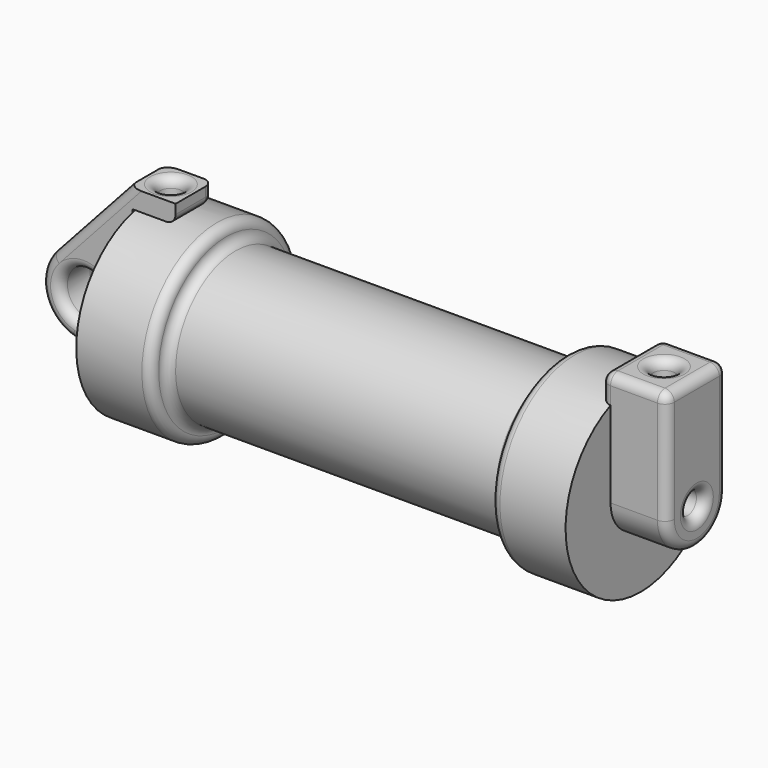
from build123d import *

# Parameters (mm, degrees)
F0_W            = 5.842
F0_H            = 12.7
F0_R            = 3.175
F2_DEPTH        = 3.175
F3_R            = 1.524
F4_DEPTH        = 7.62
F4_DEPTH_BACK   = 1.27
F5_DEPTH        = 56.134
F6_R            = 1.524
F7_DEPTH        = 10.414
F8_R            = 1.524
F9_DEPTH        = 17.78
F10_F1_R        = 1.27
F10_F2_R        = 1.2699
F10_2_T1_DEPTH  = 18.5821257943
F10_2_T3_DEPTH  = 4.572
F10_2_T5_DEPTH  = 4.445
F10_2_T7_DEPTH  = 8.255
F10_2_T9_DEPTH  = 17.7294216388
F10_2_S13_W     = 1.27
F10_2_S13_H     = 1.27
F10_2_T14_DEPTH = 1.27
F10_2_T20_ANGLE = 116.8111069241
F10_2_T26_ANGLE = 116.8111069241


# Not quite as in the source:
# - a fillet or chamfer that OpenCascade refuses, or shapes differently, is made with other operations: its cross-section is extruded or revolved along the edge and cut away or added
# - a fillet or chamfer is up to 0.001 mm smaller than in the source, because OpenCascade refuses the exact size


with BuildPart() as f1:
    # F0 (on Front) → F1 (revolve)
    with BuildSketch(Plane.XZ):
        with Locations((2.921, 6.35)):
            Rectangle(F0_W, F0_H)
        Polygon((5.842, 12.7), (5.842, 0), (66.294, 0), (66.294, 12.7), (56.134, 12.7), (56.134, 10.16), (10.16, 10.16), (10.16, 12.7), align=None)
    revolve(axis=Axis((33.147, 0, 0), (-1, 0, 0)))

    # F3 (on face) → F4 (join, two sides)
    with BuildSketch(Plane.YZ.offset(66.294)) as f4_sk:
        with BuildLine():
            ThreePointArc((-5.08, 0), (0, 5.08), (5.08, 0))
            Line((5.08, 0), (5.08, 11.6397422652))
            ThreePointArc((5.08, 11.6397422652), (0, 12.7), (-5.08, 11.6397422652))
            Line((-5.08, 11.6397422652), (-5.08, 0))
        make_face()
        with BuildLine():
            ThreePointArc((-5.08, 0), (0, -5.08), (5.08, 0))
            ThreePointArc((5.08, 0), (0, 5.08), (-5.08, 0))
        make_face()
        Circle(F3_R, mode=Mode.SUBTRACT)
        with BuildLine():
            ThreePointArc((-5.08, 11.6397422652), (0, 12.7), (5.08, 11.6397422652))
            Line((5.08, 11.6397422652), (5.08, 15.24))
            Line((5.08, 15.24), (-5.08, 15.24))
            Line((-5.08, 15.24), (-5.08, 11.6397422652))
        make_face()
    extrude(amount=F4_DEPTH)
    extrude(f4_sk.sketch, amount=-F4_DEPTH_BACK)

    # F3 (on face) → F5 (cut, through all)
    with BuildSketch(Plane.YZ.offset(66.294)):
        Circle(F3_R)
    extrude(amount=-F5_DEPTH, mode=Mode.SUBTRACT)

    # F6 (on face) → F7 (cut)
    with BuildSketch(Plane.XY.offset(15.24)):
        with Locations((69.469, 0)):
            Circle(F6_R)
    extrude(amount=-F7_DEPTH, mode=Mode.SUBTRACT)


with BuildPart() as f2:
    # F0 (on Front) → F2 (new body, symmetric)
    with BuildSketch(Plane.XZ):
        with BuildLine():
            Line((-0.9398, 0), (0, 0))
            Line((0, 0), (0, 12.7))
            Line((0, 12.7), (5.842, 12.7))
            Line((5.842, 12.7), (5.842, 15.24))
            Line((5.842, 15.24), (-0.508, 15.24))
            Line((-0.508, 15.24), (-10.8806298187, 3.8475430269))
            ThreePointArc((-10.8806298187, 3.8475430269), (-4.5919612295, 5.3297205562), (-0.9398, 0))
        make_face()
        with BuildLine():
            Line((5.842, 0), (0, 0))
            Line((0, 0), (-0.9398, 0))
            ThreePointArc((-0.9398, 0), (-3.1957909266, -4.5493385486), (-8.1826630726, -5.5069827884))
            Line((-8.1826630726, -5.5069827884), (5.842, -9.398))
            Line((5.842, -9.398), (5.842, 0))
        make_face()
        with BuildLine():
            ThreePointArc((-8.1826630726, -5.5069827884), (-3.1957909266, -4.5493385486), (-0.9398, 0))
            ThreePointArc((-0.9398, 0), (-4.5919612295, 5.3297205562), (-10.8806298187, 3.8475430269))
            ThreePointArc((-10.8806298187, 3.8475430269), (-12.1459778134, -1.5837270034), (-8.1826630726, -5.5069827884))
        make_face()
        with Locations((-6.6548, 0)):
            Circle(F0_R, mode=Mode.SUBTRACT)
    extrude(amount=F2_DEPTH, both=True)


with BuildPart() as f9_tool:
    # F8 (on face) → F9 (new body)
    with BuildSketch(Plane.XY.offset(15.24)):
        with Locations((2.667, 0)):
            Circle(F8_R)
    extrude(amount=-F9_DEPTH)


with BuildPart() as f1_1:
    add(f1.part)

    # F9: cut by f9_tool
    add(f9_tool.part, mode=Mode.SUBTRACT)

    # F10: fillet of radius 1.27 on 14 edges, made by hand

    # F10_f1
    f10_f1_edges = [f1_1.edges().sort_by_distance(p)[0] for p in [
        (10.16, 0, -10.16),
        (56.134, 0, -10.16),
    ]]
    fillet(f10_f1_edges, radius=F10_F1_R)

    # F10_f2 (radius 1.27 in the source; OpenCascade refuses exactly that, so slightly less here)
    f10_f2_edges = [f1_1.edges().sort_by_distance(p)[0] for p in [
        (73.914, -1.524, 0),
        (73.914, 0, -5.08),
        (65.024, 5.08, 13.4398711326),
        (65.024, 0, 15.24),
        (65.024, -5.08, 13.4398711326),
        (67.945, 0, 15.24),
        (73.914, 0, 15.24),
        (10.16, 0, -12.7),
        (56.134, 0, -12.7),
        (69.469, -5.08, 15.24),
        (69.469, 5.08, 15.24),
        (73.914, -5.08, 7.62),
        (73.914, 5.08, 7.62),
    ]]
    fillet(f10_f2_edges, radius=F10_F2_R)


with BuildPart() as f2_1:
    add(f2.part)

    # F9: cut by f9_tool
    add(f9_tool.part, mode=Mode.SUBTRACT)

    # F10#2: fillet of radius 1.27 on 10 edges, made by hand

    # F10_2_s2 → F10_2_t1 (cut)
    with BuildSketch(Plane(origin=(9.4938886236, 0, 10.4273187748), x_dir=(0, 1, 0), z_dir=(-0.6732358752, 0, -0.7394277898))):
        with BuildLine():
            ThreePointArc((3.175, -9.3657440555), (2.8030256121, -10.2637696676), (1.905, -10.6357440555))
            Line((1.905, -10.6357440555), (3.175, -10.6357440555))
            Line((3.175, -10.6357440555), (3.175, -9.3657440555))
        make_face()
        with BuildLine():
            ThreePointArc((-3.175, -9.3657440555), (-2.8030256121, -10.2637696676), (-1.905, -10.6357440555))
            Line((-1.905, -10.6357440555), (-3.175, -10.6357440555))
            Line((-3.175, -10.6357440555), (-3.175, -9.3657440555))
        make_face()
    extrude(amount=F10_2_T1_DEPTH, mode=Mode.SUBTRACT)

    # F10_2_s4 → F10_2_t3 (cut)
    with BuildSketch(Plane.YZ):
        with BuildLine():
            ThreePointArc((3.175, 13.97), (2.8030256121, 13.0719743879), (1.905, 12.7))
            Line((1.905, 12.7), (3.175, 12.7))
            Line((3.175, 12.7), (3.175, 13.97))
        make_face()
    extrude(amount=F10_2_T3_DEPTH, mode=Mode.SUBTRACT)

    # F10_2_s6 → F10_2_t5 (cut)
    with BuildSketch(Plane.XY.offset(13.97)):
        with BuildLine():
            ThreePointArc((4.572, 3.175), (5.4700256121, 2.8030256121), (5.842, 1.905))
            Line((5.842, 1.905), (5.842, 3.175))
            Line((5.842, 3.175), (4.572, 3.175))
        make_face()
    extrude(amount=F10_2_T5_DEPTH, mode=Mode.SUBTRACT)

    # F10_2_s8 → F10_2_t7 (cut)
    with BuildSketch(Plane.XZ.offset(-1.905)):
        with BuildLine():
            ThreePointArc((4.572, 12.7), (5.4700256121, 13.0719743879), (5.842, 13.97))
            Line((5.842, 13.97), (5.842, 12.7))
            Line((5.842, 12.7), (4.572, 12.7))
        make_face()
    extrude(amount=F10_2_T7_DEPTH, mode=Mode.SUBTRACT)

    # F10_2_s10 → F10_2_t9 (cut)
    with BuildSketch(Plane(origin=(-6.179167626, 0, 1.7143547379), x_dir=(0, 1, 0), z_dir=(0.9636015378, 0, -0.2673426199))):
        with BuildLine():
            ThreePointArc((-1.905, -7.4941116667), (-2.8030256121, -7.1221372788), (-3.175, -6.2241116667))
            Line((-3.175, -6.2241116667), (-3.175, -7.4941116667))
            Line((-3.175, -7.4941116667), (-1.905, -7.4941116667))
        make_face()
        with BuildLine():
            ThreePointArc((1.905, -7.4941116667), (2.8030256121, -7.1221372788), (3.175, -6.2241116667))
            Line((3.175, -6.2241116667), (3.175, -7.4941116667))
            Line((3.175, -7.4941116667), (1.905, -7.4941116667))
        make_face()
    extrude(amount=F10_2_T9_DEPTH, mode=Mode.SUBTRACT)


with BuildPart() as f10_2_tool12:
    # F10_2_s13 → F10_2_t14 (new body)
    with BuildSketch(Plane.YZ.offset(4.572)):
        with Locations((2.54, 13.335)):
            Rectangle(F10_2_S13_W, F10_2_S13_H)
    extrude(amount=F10_2_T14_DEPTH)

    # F10_2_s15 → F10_2_t16 (revolve, cut)
    with BuildSketch(Plane(origin=(4.572, 1.905, 13.97), x_dir=(0, -0.7071067812, 0.7071067812), z_dir=(0, 0.7071067812, 0.7071067812))):
        with BuildLine():
            ThreePointArc((0, -1.27), (1.27, 0), (0, 1.27))
            Line((0, 1.27), (0, -1.27))
        make_face()
    revolve(axis=Axis((4.572, 1.905, 13.97), (1, 0, 0)), mode=Mode.SUBTRACT)


with BuildPart() as f2_2:
    add(f2_1.part)

    # F10_2_t11: cut F10_2_tool12
    add(f10_2_tool12.part, mode=Mode.SUBTRACT)

    # F10_2_s17 → F10_2_t18 (revolve, cut)
    with BuildSketch(Plane.XY):
        with BuildLine():
            ThreePointArc((-2.2098, 3.175), (-3.1078256121, 2.8030256121), (-3.4798, 1.905))
            Line((-3.4798, 1.905), (-3.4798, 3.175))
            Line((-3.4798, 3.175), (-2.2098, 3.175))
        make_face()
    revolve(axis=Axis((-6.6548, 3.175, 0), (0, -1, 0)), mode=Mode.SUBTRACT)

    # F10_2_s19 → F10_2_t20 (revolve, cut)
    with BuildSketch(Plane(origin=(-3.0162650989, 0, -3.3128214309), x_dir=(0, 1, 0), z_dir=(0.6732358752, 0, 0.7394277898))):
        with BuildLine():
            ThreePointArc((3.175, 9.3657440555), (2.8030256121, 10.2637696676), (1.905, 10.6357440555))
            Line((1.905, 10.6357440555), (3.175, 10.6357440555))
            Line((3.175, 10.6357440555), (3.175, 9.3657440555))
        make_face()
    revolve(axis=Axis((-6.6548, 3.175, 0), (0, -1, 0)), revolution_arc=F10_2_T20_ANGLE, mode=Mode.SUBTRACT)

    # F10_2_s21 → F10_2_t22 (revolve, cut)
    with BuildSketch(Plane.XY):
        with BuildLine():
            ThreePointArc((-2.2098, -3.175), (-3.1078256121, -2.8030256121), (-3.4798, -1.905))
            Line((-3.4798, -1.905), (-3.4798, -3.175))
            Line((-3.4798, -3.175), (-2.2098, -3.175))
        make_face()
    revolve(axis=Axis((-6.6548, -3.175, 0), (0, -1, 0)), mode=Mode.SUBTRACT)

    # F10_2_s23 → F10_2_t24 (revolve, cut)
    with BuildSketch(Plane.XZ):
        with BuildLine():
            ThreePointArc((5.461, 15.24), (4.5629743879, 14.8680256121), (4.191, 13.97))
            Line((4.191, 13.97), (4.191, 15.24))
            Line((4.191, 15.24), (5.461, 15.24))
        make_face()
    revolve(axis=Axis((2.667, 0, 15.24), (0, 0, 1)), mode=Mode.SUBTRACT)

    # F10_2_s25 → F10_2_t26 (revolve, cut)
    with BuildSketch(Plane(origin=(-3.0162650989, 0, -3.3128214309), x_dir=(0, 1, 0), z_dir=(0.6732358752, 0, 0.7394277898))):
        with BuildLine():
            ThreePointArc((-3.175, 9.3657440555), (-2.8030256121, 10.2637696676), (-1.905, 10.6357440555))
            Line((-1.905, 10.6357440555), (-3.175, 10.6357440555))
            Line((-3.175, 10.6357440555), (-3.175, 9.3657440555))
        make_face()
    revolve(axis=Axis((-6.6548, -3.175, 0), (0, -1, 0)), revolution_arc=F10_2_T26_ANGLE, mode=Mode.SUBTRACT)


solid = Compound([f1_1.part, f2_2.part])
